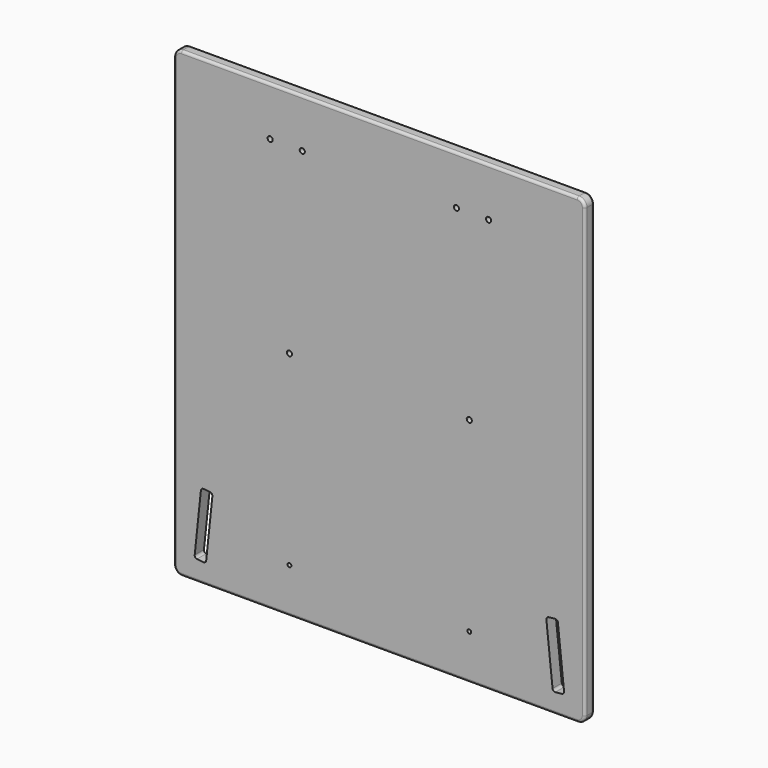
from build123d import *

# Parameters (mm, degrees)
F0_W           = 320
F0_H           = 360
F1_DEPTH       = 9
F3_DEPTH       = 9.001
F4_R           = 2
F5_R           = 6
F7_D           = 3
F7_CSINK_D     = 5
F7_CSINK_ANGLE = 90
F9_D           = 4
F10_R          = 2


# Not quite as in the source:
# - a pattern or mirror of a feature is missing from the dataset's text; its kind, count and spacing are read off the source's solid
# - a feature names something its author has since deleted; it is built from what else it names


with BuildPart() as f1:
    # F0 (on Front) → F1 (new body)
    with BuildSketch(Plane.XZ):
        with Locations((0, 180)):
            Rectangle(F0_W, F0_H)
    extrude(amount=-F1_DEPTH)

    # F2 (on Front) → F3 (cut, through all)
    with BuildSketch(Plane.XZ):
        Polygon((-129.7735768366, 64.7260947684), (-138.7242738949, 65.6668509378), (-143.9506970583, 15.9407561694), (-135, 15), align=None)
    f3 = extrude(amount=-F3_DEPTH, mode=Mode.SUBTRACT)

    # F3_copies: F3 across plane
    add(f3.mirror(Plane(origin=(0, 0, 0), x_dir=(0, 0, 1), z_dir=(1, 0, 0))), mode=Mode.SUBTRACT)

    # F4
    f4_edges = [f1.edges().sort_by_distance(p)[0] for p in [
        (-135, 4.5, 15),
        (-143.950697, 4.5, 15.940756),
        (-129.773577, 4.5, 64.726095),
        (-138.724274, 4.5, 65.666851),
    ]]
    fillet(f4_edges, radius=F4_R)

    # F5
    f5_edges = [f1.edges().sort_by_distance(p)[0] for p in [
        (160, 4.5, 0),
        (160, 4.5, 360),
        (-160, 4.5, 360),
        (-160, 4.5, 0),
    ]]
    fillet(f5_edges, radius=F5_R)

    # F7 (through all)
    with Locations(Plane(origin=(0, 9, 0), x_dir=(-1, 0, 0), z_dir=(0, 1, 0))):
        with Locations((-70, 35), (70, 35)):
            CounterSinkHole(F7_D / 2, F7_CSINK_D / 2, counter_sink_angle=F7_CSINK_ANGLE)

    # F9 (through all)
    with Locations(Plane(origin=(0, 9, 0), x_dir=(-1, 0, 0), z_dir=(0, 1, 0))):
        with Locations((-70, 180), (70, 180), (85, 322), (60, 322), (-60, 322), (-85, 322)):
            Hole(F9_D / 2)

    # F10
    f10_edges = [f1.edges().sort_by_distance(p)[0] for p in [
        (160, 9, 180),
        (160, 0, 180),
        (0, 0, 360),
        (158.242641, 0, 358.242641),
        (-158.242641, 0, 358.242641),
        (-160, 0, 180),
        (158.242641, 0, 1.757359),
        (-158.242641, 0, 1.757359),
        (0, 0, 0),
        (0, 9, 360),
        (158.242641, 9, 358.242641),
        (-158.242641, 9, 358.242641),
        (-160, 9, 180),
        (158.242641, 9, 1.757359),
        (-158.242641, 9, 1.757359),
        (0, 9, 0),
        (143.950697, 4.5, 15.940756),
        (138.724274, 4.5, 65.666851),
        (129.773577, 4.5, 64.726095),
        (135, 4.5, 15),
    ]]
    fillet(f10_edges, radius=F10_R)


solid = f1.part
